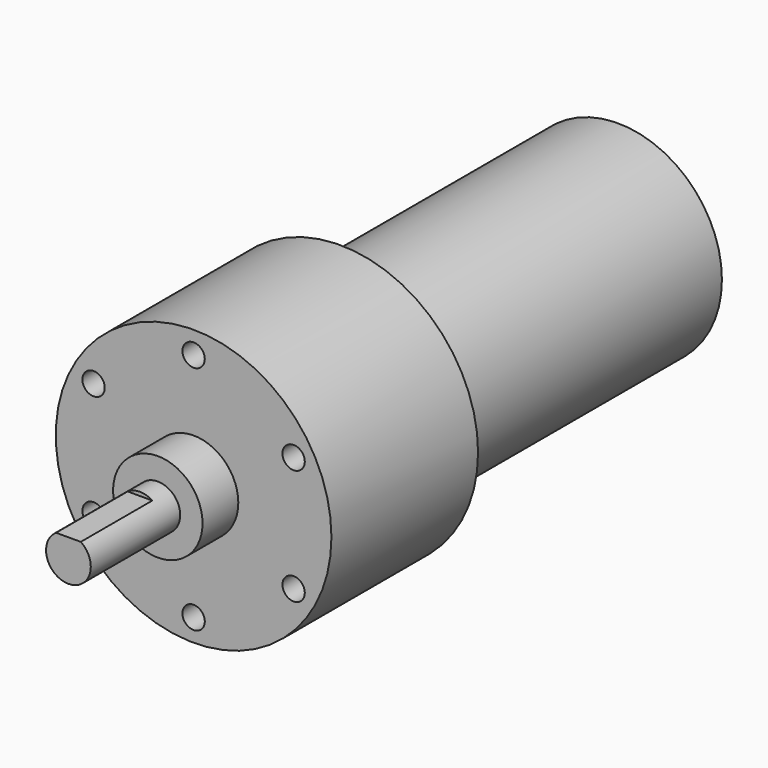
from build123d import *

# Parameters (mm, degrees)
F0_R             = 13.95
F1_DEPTH         = 46.6
F2_R             = 18.5
F2_R_2           = 13.95
F3_DEPTH         = 24.6
F4_R             = 6
F5_DEPTH         = 6
F6_R             = 3
F7_DEPTH         = 15
F9_DEPTH         = 12
F10_R            = 1.5
F11_DEPTH        = 3.4
F11_COPIES_COUNT = 6


# Not quite as in the source:
# - a pattern or mirror of a feature is missing from the dataset's text; its kind, count and spacing are read off the source's solid


with BuildPart() as f1:
    # F0 (on Front) → F1 (new body)
    with BuildSketch(Plane.XZ):
        Circle(F0_R)
    extrude(amount=F1_DEPTH)

    # F2 (on face) → F3 (join)
    with BuildSketch(Plane.XZ.offset(46.6)):
        Circle(F2_R)
        Circle(F2_R_2, mode=Mode.SUBTRACT)
        Circle(F2_R_2)
    extrude(amount=F3_DEPTH)

    # F4 (on face) → F5 (join)
    with BuildSketch(Plane.XZ.offset(71.2)):
        Circle(F4_R)
    extrude(amount=F5_DEPTH)

    # F6 (on face) → F7 (join)
    with BuildSketch(Plane.XZ.offset(77.2)):
        Circle(F6_R)
    extrude(amount=F7_DEPTH)

    # F8 (on face) → F9 (cut)
    with BuildSketch(Plane.XZ.offset(92.2)):
        with BuildLine():
            Line((-6.2269931659, 8.3767892187), (-6.2269931659, 2.5))
            Line((-6.2269931659, 2.5), (-1.6583123952, 2.5))
            ThreePointArc((-1.6583123952, 2.5), (0, 3), (1.6583123952, 2.5))
            Line((1.6583123952, 2.5), (9.3986019492, 2.5))
            Line((9.3986019492, 2.5), (9.3986019492, 8.3767892187))
            Line((9.3986019492, 8.3767892187), (-6.2269931659, 8.3767892187))
        make_face()
        with BuildLine():
            ThreePointArc((1.6583123952, 2.5), (0, 3), (-1.6583123952, 2.5))
            Line((-1.6583123952, 2.5), (1.6583123952, 2.5))
        make_face()
    extrude(amount=-F9_DEPTH, mode=Mode.SUBTRACT)

    # F10 (on face) → F11 (cut)
    with BuildSketch(Plane.XZ.offset(71.2)):
        with Locations((0, 15.5)):
            Circle(F10_R)
    f11 = extrude(amount=-F11_DEPTH, mode=Mode.SUBTRACT)

    # F11_copies: F11 ×6 about axis
    f11_copies_axis = Axis((0, 0, 0), (0, 1, 0))
    for i in range(1, F11_COPIES_COUNT):
        add(f11.rotate(f11_copies_axis, i * 360 / F11_COPIES_COUNT), mode=Mode.SUBTRACT)


solid = f1.part
